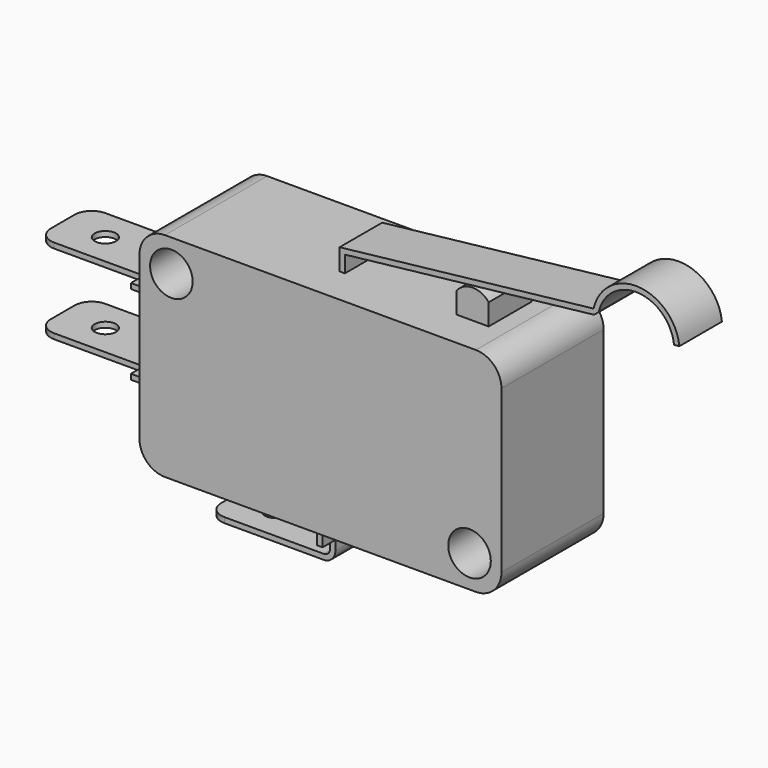
from build123d import *

# Parameters (mm, degrees)
F0_W      = 26.9875
F0_H      = 15.875
F1_DEPTH  = 4.7625
F3_DEPTH  = 1.984375
F5_DEPTH  = 3.96875
F7_DEPTH  = 1.984375
F8_W      = 9.525
F8_H      = 0.396875
F9_DEPTH  = 2.38125
F10_W     = 1.5875
F10_H     = 7.14375
F11_DEPTH = 0.396875
F12_R     = 0.79375
F13_DEPTH = 11.1135
F14_R     = 1.27
F16_DEPTH = 2.38125
F17_W     = 7.14375
F17_H     = 1.5875
F18_DEPTH = 0.396875
F19_R     = 0.79375
F20_DEPTH = 0.396875
F21_R     = 1.27
F22_R     = 1.5875
F23_DEPTH = 9.526
F24_R     = 1.5875
F25_DEPTH = 9.526
F26_R     = 1.905


# Not quite as in the source:
# - a pattern or mirror of a feature is missing from the dataset's text; its kind, count and spacing are read off the source's solid


with BuildPart() as f1:
    # F0 (on Front) → F1 (new body, symmetric)
    with BuildSketch(Plane.XZ):
        Rectangle(F0_W, F0_H)
    extrude(amount=F1_DEPTH, both=True)

    # F2 (on Front) → F3 (join, symmetric)
    with BuildSketch(Plane.XZ):
        Polygon((-0.79375, 9.525), (-0.79375, 7.9375), (-0.396875, 7.9375), (-0.396875, 9.1702745369), (18.1811773834, 11.260551947), (18.136803665, 11.6549384817), align=None)
    extrude(amount=F3_DEPTH, both=True)

    # F4 (on face) → F5 (join, through all)
    with BuildSketch(Plane.XZ.offset(1.984375)):
        with BuildLine():
            Line((24.1364444602, 11.2193732511), (24.5311773834, 11.260551947))
            ThreePointArc((24.5311773834, 11.260551947), (21.5009714287, 14.1650848753), (18.136803665, 11.6549384817))
            Line((18.136803665, 11.6549384817), (18.1811773834, 11.260551947))
            Line((18.1811773834, 11.260551947), (18.5234844717, 11.5655644399))
            ThreePointArc((18.5234844717, 11.5655644399), (21.4765397487, 13.7689625979), (24.1364444602, 11.2193732511))
        make_face()
    extrude(amount=-F5_DEPTH)

    # F6 (on Front) → F7 (join, symmetric)
    with BuildSketch(Plane.XZ):
        with BuildLine():
            Line((7.9375, 7.9375), (10.31875, 7.9375))
            Line((10.31875, 7.9375), (10.31875, 9.525))
            ThreePointArc((10.31875, 9.525), (9.128125, 10.0965), (7.9375, 9.525))
            Line((7.9375, 9.525), (7.9375, 7.9375))
        make_face()
    extrude(amount=F7_DEPTH, both=True)

    # F8 (on Front) → F9 (join, symmetric)
    with BuildSketch(Plane.XZ):
        with Locations((-18.25625, 2.9765625)):
            Rectangle(F8_W, F8_H)
    f9 = extrude(amount=F9_DEPTH, both=True)

    # F9_copies: F9 across plane
    add(f9.mirror(Plane(origin=(0, 0, 0), x_dir=(-1, 0, 0), z_dir=(0, 0, -1))))

    # F10 (on face) → F11 (join, through all)
    with BuildSketch(Plane.XY.offset(3.175)):
        with Locations((-14.2875, 0)):
            Rectangle(F10_W, F10_H)
    f11 = extrude(amount=-F11_DEPTH)

    # F11_copies: F11 across plane
    add(f11.mirror(Plane(origin=(0, 0, 0), x_dir=(-1, 0, 0), z_dir=(0, 0, -1))))

    # F12 (on face) → F13 (cut, through all)
    with BuildSketch(Plane.XY.offset(3.175)):
        with Locations((-19.84375, 0)):
            Circle(F12_R)
    extrude(amount=-F13_DEPTH, mode=Mode.SUBTRACT)

    # F14
    f14_edges = [f1.edges().sort_by_distance(p)[0] for p in [
        (-23.01875, -2.38125, 2.976562),
        (-23.01875, 2.38125, 2.976562),
    ]]
    fillet(f14_edges, radius=F14_R)

    # F15 (on Front) → F16 (join, symmetric)
    with BuildSketch(Plane.XZ):
        with BuildLine():
            Line((-0.79375, -10.2451657598), (-0.79375, -7.9375))
            Line((-0.79375, -7.9375), (-1.190625, -7.9375))
            Line((-1.190625, -7.9375), (-1.190625, -10.2451657598))
            ThreePointArc((-1.190625, -10.2451657598), (-1.3284193212, -10.5778306788), (-1.6610842402, -10.715625))
            Line((-1.6610842402, -10.715625), (-10.31875, -10.715625))
            Line((-10.31875, -10.715625), (-10.31875, -11.1125))
            Line((-10.31875, -11.1125), (-1.6610842402, -11.1125))
            ThreePointArc((-1.6610842402, -11.1125), (-1.0477863174, -10.8584636826), (-0.79375, -10.2451657598))
        make_face()
    extrude(amount=F16_DEPTH, both=True)

    # F17 (on face) → F18 (join, through all)
    with BuildSketch(Plane(origin=(-1.190625, 0, 0), x_dir=(0, -1, 0), z_dir=(-1, 0, 0))):
        with Locations((0, -8.73125)):
            Rectangle(F17_W, F17_H)
    extrude(amount=-F18_DEPTH)

    # F19 (on face) → F20 (cut, through all)
    with BuildSketch(Plane(origin=(0, 0, -11.1125), x_dir=(1, 0, 0), z_dir=(0, 0, -1))):
        with Locations((-7.14375, 0)):
            Circle(F19_R)
    extrude(amount=-F20_DEPTH, mode=Mode.SUBTRACT)

    # F21
    f21_edges = [f1.edges().sort_by_distance(p)[0] for p in [
        (-10.31875, 2.38125, -10.914062),
        (-10.31875, -2.38125, -10.914062),
        (-23.01875, 2.38125, -2.976562),
        (-23.01875, -2.38125, -2.976562),
    ]]
    fillet(f21_edges, radius=F21_R)

    # F22 (on face) → F23 (cut, through all)
    with BuildSketch(Plane.XZ.offset(4.7625)):
        with Locations((-11.1125, 5.55625)):
            Circle(F22_R)
    extrude(amount=-F23_DEPTH, mode=Mode.SUBTRACT)

    # F24 (on face) → F25 (cut, through all)
    with BuildSketch(Plane.XZ.offset(4.7625)):
        with Locations((11.1125, -5.55625)):
            Circle(F24_R)
    extrude(amount=-F25_DEPTH, mode=Mode.SUBTRACT)

    # F26
    f26_edges = [f1.edges().sort_by_distance(p)[0] for p in [
        (-13.49375, 0, 7.9375),
        (13.49375, 0, 7.9375),
        (13.49375, 0, -7.9375),
        (-13.49375, 0, -7.9375),
    ]]
    fillet(f26_edges, radius=F26_R)


solid = f1.part
